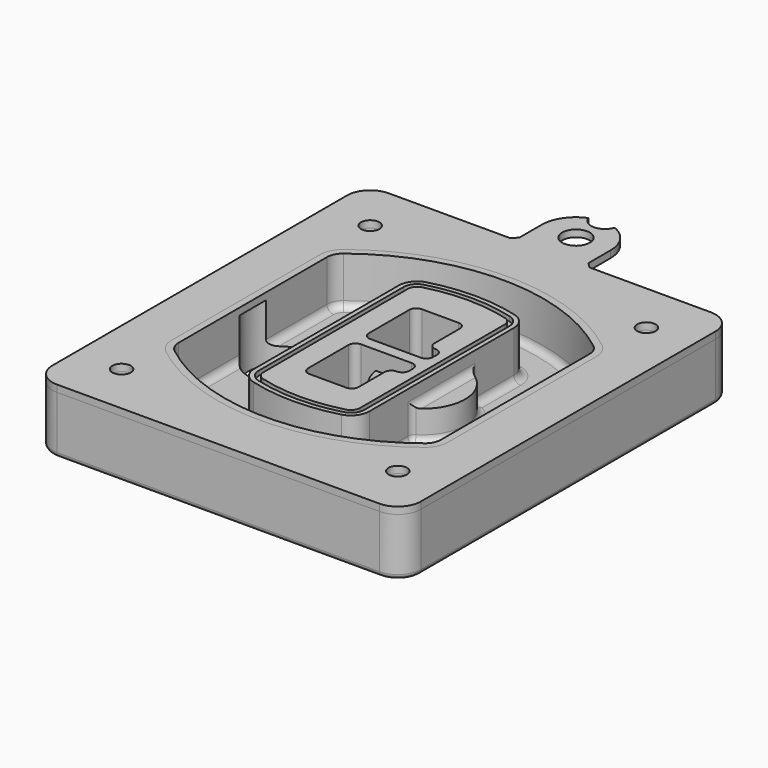
from build123d import *

# Parameters (mm, degrees)
F0_R      = 4
F1_DEPTH  = 25
F2_DEPTH  = 3
F3_DEPTH  = 18
F5_DEPTH  = 21
F6_DEPTH  = 2
F8_DEPTH  = 20
F9_DEPTH  = 16
F10_DEPTH = 25
F7_R      = 6
F7_R_2    = 4
F11_DEPTH = 6
F13_DEPTH = 9
F14_R     = 3
F15_R     = 2
F16_R     = 6
F16_R_2   = 4
F17_DEPTH = 3


with BuildPart() as f1:
    # F0 (on Top) → F1 (new body)
    with BuildSketch(Plane.XY):
        with BuildLine():
            ThreePointArc((-80, -80), (-77.0710678119, -87.0710678119), (-70, -90))
            Line((-70, -90), (70, -90))
            ThreePointArc((70, -90), (77.0710678119, -87.0710678119), (80, -80))
            Line((80, -80), (80, 80))
            ThreePointArc((80, 80), (77.0710678119, 87.0710678119), (70, 90))
            Line((70, 90), (-70, 90))
            ThreePointArc((-70, 90), (-77.0710678119, 87.0710678119), (-80, 80))
            Line((-80, 80), (-80, -80))
        make_face()
        with Locations((-60, -67.5)):
            Circle(F0_R, mode=Mode.SUBTRACT)
        with Locations((60, -67.5)):
            Circle(F0_R, mode=Mode.SUBTRACT)
        with Locations((-60, 67.5)):
            Circle(F0_R, mode=Mode.SUBTRACT)
        with BuildLine():
            ThreePointArc((-64, 40.2934422872), (-62.5820384798, 46.4328484224), (-58.6153846154, 51.3286200352))
            ThreePointArc((-58.6153846154, 51.3286200352), (0, 71.5), (58.6153846154, 51.3286200352))
            ThreePointArc((58.6153846154, 51.3286200352), (62.5820384798, 46.4328484224), (64, 40.2934422872))
            Line((64, 40.2934422872), (64, -40.2934422872))
            ThreePointArc((64, -40.2934422872), (62.5820384798, -46.4328484224), (58.6153846154, -51.3286200352))
            ThreePointArc((58.6153846154, -51.3286200352), (0, -71.5), (-58.6153846154, -51.3286200352))
            ThreePointArc((-58.6153846154, -51.3286200352), (-62.5820384798, -46.4328484224), (-64, -40.2934422872))
            Line((-64, -40.2934422872), (-64, 40.2934422872))
        make_face(mode=Mode.SUBTRACT)
        with Locations((60, 67.5)):
            Circle(F0_R, mode=Mode.SUBTRACT)
        with BuildLine():
            ThreePointArc((58.6153846154, 51.3286200352), (0, 71.5), (-58.6153846154, 51.3286200352))
            ThreePointArc((-58.6153846154, 51.3286200352), (-62.5820384798, 46.4328484224), (-64, 40.2934422872))
            Line((-64, 40.2934422872), (-64, -40.2934422872))
            ThreePointArc((-64, -40.2934422872), (-62.5820384798, -46.4328484224), (-58.6153846154, -51.3286200352))
            ThreePointArc((-58.6153846154, -51.3286200352), (0, -71.5), (58.6153846154, -51.3286200352))
            ThreePointArc((58.6153846154, -51.3286200352), (62.5820384798, -46.4328484224), (64, -40.2934422872))
            Line((64, -40.2934422872), (64, 40.2934422872))
            ThreePointArc((64, 40.2934422872), (62.5820384798, 46.4328484224), (58.6153846154, 51.3286200352))
        make_face()
        with BuildLine():
            Line((-60, -40.2934422872), (-60, 40.2934422872))
            ThreePointArc((-60, 40.2934422872), (-58.9871703427, 44.6787323838), (-56.1538461538, 48.1757121072))
            ThreePointArc((-56.1538461538, 48.1757121072), (0, 67.5), (56.1538461538, 48.1757121072))
            ThreePointArc((56.1538461538, 48.1757121072), (58.9871703427, 44.6787323838), (60, 40.2934422872))
            Line((60, 40.2934422872), (60, -40.2934422872))
            ThreePointArc((60, -40.2934422872), (58.9871703427, -44.6787323838), (56.1538461538, -48.1757121072))
            ThreePointArc((56.1538461538, -48.1757121072), (0, -67.5), (-56.1538461538, -48.1757121072))
            ThreePointArc((-56.1538461538, -48.1757121072), (-58.9871703427, -44.6787323838), (-60, -40.2934422872))
        make_face(mode=Mode.SUBTRACT)
        with BuildLine():
            ThreePointArc((-56.1538461538, 48.1757121072), (-58.9871703427, 44.6787323838), (-60, 40.2934422872))
            Line((-60, 40.2934422872), (-60, -40.2934422872))
            ThreePointArc((-60, -40.2934422872), (-58.9871703427, -44.6787323838), (-56.1538461538, -48.1757121072))
            ThreePointArc((-56.1538461538, -48.1757121072), (0, -67.5), (56.1538461538, -48.1757121072))
            ThreePointArc((56.1538461538, -48.1757121072), (58.9871703427, -44.6787323838), (60, -40.2934422872))
            Line((60, -40.2934422872), (60, 40.2934422872))
            ThreePointArc((60, 40.2934422872), (58.9871703427, 44.6787323838), (56.1538461538, 48.1757121072))
            ThreePointArc((56.1538461538, 48.1757121072), (0, 67.5), (-56.1538461538, 48.1757121072))
        make_face()
        with BuildLine():
            ThreePointArc((54.3076923077, 45.8110311612), (56.2910192399, 43.3631453548), (57, 40.2934422872))
            Line((57, 40.2934422872), (57, -40.2934422872))
            ThreePointArc((57, -40.2934422872), (56.2910192399, -43.3631453548), (54.3076923077, -45.8110311612))
            ThreePointArc((54.3076923077, -45.8110311612), (0, -64.5), (-54.3076923077, -45.8110311612))
            ThreePointArc((-54.3076923077, -45.8110311612), (-56.2910192399, -43.3631453548), (-57, -40.2934422872))
            Line((-57, -40.2934422872), (-57, 40.2934422872))
            ThreePointArc((-57, 40.2934422872), (-56.2910192399, 43.3631453548), (-54.3076923077, 45.8110311612))
            ThreePointArc((-54.3076923077, 45.8110311612), (0, 64.5), (54.3076923077, 45.8110311612))
        make_face(mode=Mode.SUBTRACT)
        with BuildLine():
            Line((57, -40.2934422872), (57, 40.2934422872))
            ThreePointArc((57, 40.2934422872), (56.2910192399, 43.3631453548), (54.3076923077, 45.8110311612))
            ThreePointArc((54.3076923077, 45.8110311612), (0, 64.5), (-54.3076923077, 45.8110311612))
            ThreePointArc((-54.3076923077, 45.8110311612), (-56.2910192399, 43.3631453548), (-57, 40.2934422872))
            Line((-57, 40.2934422872), (-57, -40.2934422872))
            ThreePointArc((-57, -40.2934422872), (-56.2910192399, -43.3631453548), (-54.3076923077, -45.8110311612))
            ThreePointArc((-54.3076923077, -45.8110311612), (0, -64.5), (54.3076923077, -45.8110311612))
            ThreePointArc((54.3076923077, -45.8110311612), (56.2910192399, -43.3631453548), (57, -40.2934422872))
        make_face()
    extrude(amount=-F1_DEPTH)

    # F0 (on Top) → F2 (join)
    with BuildSketch(Plane.XY):
        with BuildLine():
            ThreePointArc((-56.1538461538, 48.1757121072), (-58.9871703427, 44.6787323838), (-60, 40.2934422872))
            Line((-60, 40.2934422872), (-60, -40.2934422872))
            ThreePointArc((-60, -40.2934422872), (-58.9871703427, -44.6787323838), (-56.1538461538, -48.1757121072))
            ThreePointArc((-56.1538461538, -48.1757121072), (0, -67.5), (56.1538461538, -48.1757121072))
            ThreePointArc((56.1538461538, -48.1757121072), (58.9871703427, -44.6787323838), (60, -40.2934422872))
            Line((60, -40.2934422872), (60, 40.2934422872))
            ThreePointArc((60, 40.2934422872), (58.9871703427, 44.6787323838), (56.1538461538, 48.1757121072))
            ThreePointArc((56.1538461538, 48.1757121072), (0, 67.5), (-56.1538461538, 48.1757121072))
        make_face()
        with BuildLine():
            ThreePointArc((54.3076923077, 45.8110311612), (56.2910192399, 43.3631453548), (57, 40.2934422872))
            Line((57, 40.2934422872), (57, -40.2934422872))
            ThreePointArc((57, -40.2934422872), (56.2910192399, -43.3631453548), (54.3076923077, -45.8110311612))
            ThreePointArc((54.3076923077, -45.8110311612), (0, -64.5), (-54.3076923077, -45.8110311612))
            ThreePointArc((-54.3076923077, -45.8110311612), (-56.2910192399, -43.3631453548), (-57, -40.2934422872))
            Line((-57, -40.2934422872), (-57, 40.2934422872))
            ThreePointArc((-57, 40.2934422872), (-56.2910192399, 43.3631453548), (-54.3076923077, 45.8110311612))
            ThreePointArc((-54.3076923077, 45.8110311612), (0, 64.5), (54.3076923077, 45.8110311612))
        make_face(mode=Mode.SUBTRACT)
    extrude(amount=F2_DEPTH)

    # F0 (on Top) → F3 (cut)
    with BuildSketch(Plane.XY):
        with BuildLine():
            Line((57, -40.2934422872), (57, 40.2934422872))
            ThreePointArc((57, 40.2934422872), (56.2910192399, 43.3631453548), (54.3076923077, 45.8110311612))
            ThreePointArc((54.3076923077, 45.8110311612), (0, 64.5), (-54.3076923077, 45.8110311612))
            ThreePointArc((-54.3076923077, 45.8110311612), (-56.2910192399, 43.3631453548), (-57, 40.2934422872))
            Line((-57, 40.2934422872), (-57, -40.2934422872))
            ThreePointArc((-57, -40.2934422872), (-56.2910192399, -43.3631453548), (-54.3076923077, -45.8110311612))
            ThreePointArc((-54.3076923077, -45.8110311612), (0, -64.5), (54.3076923077, -45.8110311612))
            ThreePointArc((54.3076923077, -45.8110311612), (56.2910192399, -43.3631453548), (57, -40.2934422872))
        make_face()
    extrude(amount=-F3_DEPTH, mode=Mode.SUBTRACT)

    # F4 (on face) → F5 (join, through all)
    with BuildSketch(Plane.XY.offset(3)):
        with BuildLine():
            ThreePointArc((-25, -39.2465276821), (-23.3511545998, -44.1109737193), (-19.0842911877, -46.9702398883))
            ThreePointArc((-19.0842911877, -46.9702398883), (0, -49.5), (19.0842911877, -46.9702398883))
            ThreePointArc((19.0842911877, -46.9702398883), (23.3511545998, -44.1109737193), (25, -39.2465276821))
            Line((25, -39.2465276821), (25, 39.2465276821))
            ThreePointArc((25, 39.2465276821), (23.3511545998, 44.1109737193), (19.0842911877, 46.9702398883))
            ThreePointArc((19.0842911877, 46.9702398883), (0, 49.5), (-19.0842911877, 46.9702398883))
            ThreePointArc((-19.0842911877, 46.9702398883), (-23.3511545998, 44.1109737193), (-25, 39.2465276821))
            Line((-25, 39.2465276821), (-25, -39.2465276821))
        make_face()
        with BuildLine():
            ThreePointArc((18.5632183908, 45.0393118368), (21.7633659499, 42.89486221), (23, 39.2465276821))
            Line((23, 39.2465276821), (23, -39.2465276821))
            ThreePointArc((23, -39.2465276821), (21.7633659499, -42.89486221), (18.5632183908, -45.0393118368))
            ThreePointArc((18.5632183908, -45.0393118368), (0, -47.5), (-18.5632183908, -45.0393118368))
            ThreePointArc((-18.5632183908, -45.0393118368), (-21.7633659499, -42.89486221), (-23, -39.2465276821))
            Line((-23, -39.2465276821), (-23, 39.2465276821))
            ThreePointArc((-23, 39.2465276821), (-21.7633659499, 42.89486221), (-18.5632183908, 45.0393118368))
            ThreePointArc((-18.5632183908, 45.0393118368), (0, 47.5), (18.5632183908, 45.0393118368))
        make_face(mode=Mode.SUBTRACT)
        with BuildLine():
            Line((23, -39.2465276821), (23, 39.2465276821))
            ThreePointArc((23, 39.2465276821), (21.7633659499, 42.89486221), (18.5632183908, 45.0393118368))
            ThreePointArc((18.5632183908, 45.0393118368), (0, 47.5), (-18.5632183908, 45.0393118368))
            ThreePointArc((-18.5632183908, 45.0393118368), (-21.7633659499, 42.89486221), (-23, 39.2465276821))
            Line((-23, 39.2465276821), (-23, -39.2465276821))
            ThreePointArc((-23, -39.2465276821), (-21.7633659499, -42.89486221), (-18.5632183908, -45.0393118368))
            ThreePointArc((-18.5632183908, -45.0393118368), (0, -47.5), (18.5632183908, -45.0393118368))
            ThreePointArc((18.5632183908, -45.0393118368), (21.7633659499, -42.89486221), (23, -39.2465276821))
        make_face()
        with BuildLine():
            ThreePointArc((18.0421455939, 43.1083837852), (20.1755772999, 41.6787507007), (21, 39.2465276821))
            Line((21, 39.2465276821), (21, -39.2465276821))
            ThreePointArc((21, -39.2465276821), (20.1755772999, -41.6787507007), (18.0421455939, -43.1083837852))
            ThreePointArc((18.0421455939, -43.1083837852), (0, -45.5), (-18.0421455939, -43.1083837852))
            ThreePointArc((-18.0421455939, -43.1083837852), (-20.1755772999, -41.6787507007), (-21, -39.2465276821))
            Line((-21, -39.2465276821), (-21, 39.2465276821))
            ThreePointArc((-21, 39.2465276821), (-20.1755772999, 41.6787507007), (-18.0421455939, 43.1083837852))
            ThreePointArc((-18.0421455939, 43.1083837852), (0, 45.5), (18.0421455939, 43.1083837852))
        make_face(mode=Mode.SUBTRACT)
        with BuildLine():
            Line((21, -39.2465276821), (21, 39.2465276821))
            ThreePointArc((21, 39.2465276821), (20.1755772999, 41.6787507007), (18.0421455939, 43.1083837852))
            ThreePointArc((18.0421455939, 43.1083837852), (0, 45.5), (-18.0421455939, 43.1083837852))
            ThreePointArc((-18.0421455939, 43.1083837852), (-20.1755772999, 41.6787507007), (-21, 39.2465276821))
            Line((-21, 39.2465276821), (-21, -39.2465276821))
            ThreePointArc((-21, -39.2465276821), (-20.1755772999, -41.6787507007), (-18.0421455939, -43.1083837852))
            ThreePointArc((-18.0421455939, -43.1083837852), (0, -45.5), (18.0421455939, -43.1083837852))
            ThreePointArc((18.0421455939, -43.1083837852), (20.1755772999, -41.6787507007), (21, -39.2465276821))
        make_face()
        with BuildLine():
            Line((-8, -2.5), (14, -2.5))
            ThreePointArc((14, -2.5), (16.1213203436, -3.3786796564), (17, -5.5))
            Line((17, -5.5), (17, -7.5))
            ThreePointArc((17, -7.5), (16.1213203436, -9.6213203436), (14, -10.5))
            ThreePointArc((14, -10.5), (11.8786796564, -11.3786796564), (11, -13.5))
            Line((11, -13.5), (11, -27.5))
            ThreePointArc((11, -27.5), (10.1213203436, -29.6213203436), (8, -30.5))
            Line((8, -30.5), (-8, -30.5))
            ThreePointArc((-8, -30.5), (-10.1213203436, -29.6213203436), (-11, -27.5))
            Line((-11, -27.5), (-11, -5.5))
            ThreePointArc((-11, -5.5), (-10.1213203436, -3.3786796564), (-8, -2.5))
        make_face(mode=Mode.SUBTRACT)
        with BuildLine():
            ThreePointArc((-8, 2.5), (-10.1213203436, 3.3786796564), (-11, 5.5))
            Line((-11, 5.5), (-11, 27.5))
            ThreePointArc((-11, 27.5), (-10.1213203436, 29.6213203436), (-8, 30.5))
            Line((-8, 30.5), (8, 30.5))
            ThreePointArc((8, 30.5), (10.1213203436, 29.6213203436), (11, 27.5))
            Line((11, 27.5), (11, 13.5))
            ThreePointArc((11, 13.5), (11.8786796564, 11.3786796564), (14, 10.5))
            ThreePointArc((14, 10.5), (16.1213203436, 9.6213203436), (17, 7.5))
            Line((17, 7.5), (17, 5.5))
            ThreePointArc((17, 5.5), (16.1213203436, 3.3786796564), (14, 2.5))
            Line((14, 2.5), (-8, 2.5))
        make_face(mode=Mode.SUBTRACT)
    extrude(amount=-F5_DEPTH)

    # F4 (on face) → F6 (cut)
    with BuildSketch(Plane.XY.offset(3)):
        with BuildLine():
            Line((23, -39.2465276821), (23, 39.2465276821))
            ThreePointArc((23, 39.2465276821), (21.7633659499, 42.89486221), (18.5632183908, 45.0393118368))
            ThreePointArc((18.5632183908, 45.0393118368), (0, 47.5), (-18.5632183908, 45.0393118368))
            ThreePointArc((-18.5632183908, 45.0393118368), (-21.7633659499, 42.89486221), (-23, 39.2465276821))
            Line((-23, 39.2465276821), (-23, -39.2465276821))
            ThreePointArc((-23, -39.2465276821), (-21.7633659499, -42.89486221), (-18.5632183908, -45.0393118368))
            ThreePointArc((-18.5632183908, -45.0393118368), (0, -47.5), (18.5632183908, -45.0393118368))
            ThreePointArc((18.5632183908, -45.0393118368), (21.7633659499, -42.89486221), (23, -39.2465276821))
        make_face()
        with BuildLine():
            ThreePointArc((18.0421455939, 43.1083837852), (20.1755772999, 41.6787507007), (21, 39.2465276821))
            Line((21, 39.2465276821), (21, -39.2465276821))
            ThreePointArc((21, -39.2465276821), (20.1755772999, -41.6787507007), (18.0421455939, -43.1083837852))
            ThreePointArc((18.0421455939, -43.1083837852), (0, -45.5), (-18.0421455939, -43.1083837852))
            ThreePointArc((-18.0421455939, -43.1083837852), (-20.1755772999, -41.6787507007), (-21, -39.2465276821))
            Line((-21, -39.2465276821), (-21, 39.2465276821))
            ThreePointArc((-21, 39.2465276821), (-20.1755772999, 41.6787507007), (-18.0421455939, 43.1083837852))
            ThreePointArc((-18.0421455939, 43.1083837852), (0, 45.5), (18.0421455939, 43.1083837852))
        make_face(mode=Mode.SUBTRACT)
    extrude(amount=-F6_DEPTH, mode=Mode.SUBTRACT)

    # F7 (on face) → F8 (join)
    with BuildSketch(Plane(origin=(0, 0, -25), x_dir=(1, 0, 0), z_dir=(0, 0, -1))):
        with BuildLine():
            ThreePointArc((3.28842436, 0), (16.7567035675, 13.4682792075), (30.224982775, 0))
            Line((30.224982775, 0), (35.224982775, 0))
            ThreePointArc((35.224982775, 0), (16.7567035675, 18.4682792075), (-1.71157564, 0))
            Line((-1.71157564, 0), (3.28842436, 0))
        make_face()
        with BuildLine():
            Line((3.28842436, 0), (30.224982775, 0))
            ThreePointArc((30.224982775, 0), (16.7567035675, 13.4682792075), (3.28842436, 0))
        make_face()
        with BuildLine():
            ThreePointArc((3.28842436, 0), (16.7567035675, -13.4682792075), (30.224982775, 0))
            Line((30.224982775, 0), (3.28842436, 0))
        make_face()
        with BuildLine():
            Line((35.224982775, 0), (30.224982775, 0))
            ThreePointArc((30.224982775, 0), (16.7567035675, -13.4682792075), (3.28842436, 0))
            Line((3.28842436, 0), (-1.71157564, 0))
            ThreePointArc((-1.71157564, 0), (16.7567035675, -18.4682792075), (35.224982775, 0))
        make_face()
    extrude(amount=-F8_DEPTH)

    # F7 (on face) → F9 (cut)
    with BuildSketch(Plane(origin=(0, 0, -25), x_dir=(1, 0, 0), z_dir=(0, 0, -1))):
        with BuildLine():
            Line((3.28842436, 0), (30.224982775, 0))
            ThreePointArc((30.224982775, 0), (16.7567035675, 13.4682792075), (3.28842436, 0))
        make_face()
        with BuildLine():
            ThreePointArc((3.28842436, 0), (16.7567035675, -13.4682792075), (30.224982775, 0))
            Line((30.224982775, 0), (3.28842436, 0))
        make_face()
    extrude(amount=-F9_DEPTH, mode=Mode.SUBTRACT)

    # F7 (on face) → F10 (cut)
    with BuildSketch(Plane(origin=(0, 0, -25), x_dir=(1, 0, 0), z_dir=(0, 0, -1))):
        with BuildLine():
            Line((-59.0318229325, 0), (-32.0952645175, 0))
            ThreePointArc((-32.0952645175, 0), (-45.563543725, 13.4682792075), (-59.0318229325, 0))
        make_face()
        with BuildLine():
            ThreePointArc((-59.0318229325, 0), (-45.563543725, -13.4682792075), (-32.0952645175, 0))
            Line((-32.0952645175, 0), (-59.0318229325, 0))
        make_face()
    extrude(amount=-F10_DEPTH, mode=Mode.SUBTRACT)

    # F7 (on face) → F11 (cut)
    with BuildSketch(Plane(origin=(0, 0, -25), x_dir=(1, 0, 0), z_dir=(0, 0, -1))):
        with Locations((60, -67.5)):
            Circle(F7_R)
        with Locations((60, -67.5)):
            Circle(F7_R_2, mode=Mode.SUBTRACT)
        with Locations((-60, -67.5)):
            Circle(F7_R)
        with Locations((-60, -67.5)):
            Circle(F7_R_2, mode=Mode.SUBTRACT)
        with Locations((-60, 67.5)):
            Circle(F7_R)
        with Locations((-60, 67.5)):
            Circle(F7_R_2, mode=Mode.SUBTRACT)
        with Locations((60, 67.5)):
            Circle(F7_R)
        with Locations((60, 67.5)):
            Circle(F7_R_2, mode=Mode.SUBTRACT)
    extrude(amount=-F11_DEPTH, mode=Mode.SUBTRACT)

    # F12 (on face) → F13 (cut, through all)
    with BuildSketch(Plane(origin=(0, 0, -9), x_dir=(1, 0, 0), z_dir=(0, 0, -1))):
        with BuildLine():
            Line((11, 13.5), (11, 17.5481537753))
            ThreePointArc((11, 17.5481537753), (2.5696536419, 11.8239143813), (-1.5415842455, 2.5))
            Line((-1.5415842455, 2.5), (3.5224848595, 2.5))
            ThreePointArc((3.5224848595, 2.5), (6.1857188154, 8.3455872281), (11.2536447004, 12.2927168648))
            ThreePointArc((11.2536447004, 12.2927168648), (11.0640958889, 12.8831798879), (11, 13.5))
        make_face()
        with BuildLine():
            ThreePointArc((11.2536447004, -12.2927168648), (6.1857188154, -8.3455872281), (3.5224848595, -2.5))
            Line((3.5224848595, -2.5), (-1.5415842455, -2.5))
            ThreePointArc((-1.5415842455, -2.5), (2.5696536419, -11.8239143813), (11, -17.5481537753))
            Line((11, -17.5481537753), (11, -13.5))
            ThreePointArc((11, -13.5), (11.0640958889, -12.8831798879), (11.2536447004, -12.2927168648))
        make_face()
        with BuildLine():
            ThreePointArc((11.2536447004, 12.2927168648), (6.1857188154, 8.3455872281), (3.5224848595, 2.5))
            Line((3.5224848595, 2.5), (14, 2.5))
            ThreePointArc((14, 2.5), (16.1213203436, 3.3786796564), (17, 5.5))
            Line((17, 5.5), (17, 7.5))
            ThreePointArc((17, 7.5), (16.1213203436, 9.6213203436), (14, 10.5))
            ThreePointArc((14, 10.5), (12.3601599782, 10.9878446101), (11.2536447004, 12.2927168648))
        make_face()
        with BuildLine():
            Line((14, -2.5), (3.5224848595, -2.5))
            ThreePointArc((3.5224848595, -2.5), (6.1857188154, -8.3455872281), (11.2536447004, -12.2927168648))
            ThreePointArc((11.2536447004, -12.2927168648), (12.3601599782, -10.9878446101), (14, -10.5))
            ThreePointArc((14, -10.5), (16.1213203436, -9.6213203436), (17, -7.5))
            Line((17, -7.5), (17, -5.5))
            ThreePointArc((17, -5.5), (16.1213203436, -3.3786796564), (14, -2.5))
        make_face()
    extrude(amount=F13_DEPTH, mode=Mode.SUBTRACT)

    # F14
    f14_edges = [f1.edges().sort_by_distance(p)[0] for p in [
        (-57, -23.703476, -18),
        (-57, 23.703476, -18),
        (25, 0, -5),
        (25, 16.526506, -11.5),
        (25, -16.526506, -11.5),
        (25, -27.886517, -18),
        (35.224983, 0, -18),
        (23.351155, -44.110974, -18),
        (0, -64.5, -18),
        (-56.291019, -43.363145, -18),
        (-56.291019, 43.363145, -18),
        (0, 64.5, -18),
        (56.291019, 43.363145, -18),
        (57, 0, -18),
        (56.291019, -43.363145, -18),
        (-23.351155, 44.110974, -18),
        (0, 49.5, -18),
        (-25, 0, -18),
        (23.351155, 44.110974, -18),
        (-23.351155, -44.110974, -18),
        (25, 27.886517, -18),
        (0, -49.5, -18),
    ]]
    fillet(f14_edges, radius=F14_R)

    # F15
    f15_edges = [f1.edges().sort_by_distance(p)[0] for p in [
        (0, -90, -25),
        (-77.071068, -87.071068, -25),
        (-80, 0, -25),
        (-77.071068, 87.071068, -25),
        (77.071068, -87.071068, -25),
        (0, 90, -25),
        (80, 0, -25),
        (77.071068, 87.071068, -25),
    ]]
    fillet(f15_edges, radius=F15_R)


with BuildPart() as f17:
    # F16 (on face) → F17 (new body, through all)
    with BuildSketch(Plane.XY):
        with BuildLine():
            ThreePointArc((5.6995065576, 118.125), (0, 114), (-5.6995065576, 118.125))
            ThreePointArc((-5.6995065576, 118.125), (-12.4597872848, 112.6018681035), (-15, 104.25))
            Line((-15, 104.25), (-15, 92.25))
            Line((-15, 92.25), (-17.25, 90))
            Line((-17.25, 90), (17.25, 90))
            Line((17.25, 90), (15, 92.25))
            Line((15, 92.25), (15, 104.25))
            ThreePointArc((15, 104.25), (12.4597872848, 112.6018681035), (5.6995065576, 118.125))
        make_face()
        with Locations((0, 104.25)):
            Circle(F16_R, mode=Mode.SUBTRACT)
        with BuildLine():
            Line((17.25, 90), (-17.25, 90))
            Line((-17.25, 90), (-70, 90))
            ThreePointArc((-70, 90), (-77.0710678119, 87.0710678119), (-80, 80))
            Line((-80, 80), (-80, -80))
            ThreePointArc((-80, -80), (-77.0710678119, -87.0710678119), (-70, -90))
            Line((-70, -90), (-17.25, -90))
            Line((-17.25, -90), (33, -90))
            Line((33, -90), (70, -90))
            ThreePointArc((70, -90), (77.0710678119, -87.0710678119), (80, -80))
            Line((80, -80), (80, 80))
            ThreePointArc((80, 80), (77.0710678119, 87.0710678119), (70, 90))
            Line((70, 90), (33, 90))
            Line((33, 90), (17.25, 90))
        make_face()
        with Locations((-60, -67.5)):
            Circle(F16_R_2, mode=Mode.SUBTRACT)
        with Locations((60, -67.5)):
            Circle(F16_R_2, mode=Mode.SUBTRACT)
        with Locations((-60, 67.5)):
            Circle(F16_R_2, mode=Mode.SUBTRACT)
        with BuildLine():
            ThreePointArc((-60, 40.2934422872), (-58.9871703427, 44.6787323838), (-56.1538461538, 48.1757121072))
            ThreePointArc((-56.1538461538, 48.1757121072), (0, 67.5), (56.1538461538, 48.1757121072))
            ThreePointArc((56.1538461538, 48.1757121072), (58.9871703427, 44.6787323838), (60, 40.2934422872))
            Line((60, 40.2934422872), (60, -40.2934422872))
            ThreePointArc((60, -40.2934422872), (58.9871703427, -44.6787323838), (56.1538461538, -48.1757121072))
            ThreePointArc((56.1538461538, -48.1757121072), (0, -67.5), (-56.1538461538, -48.1757121072))
            ThreePointArc((-56.1538461538, -48.1757121072), (-58.9871703427, -44.6787323838), (-60, -40.2934422872))
            Line((-60, -40.2934422872), (-60, 40.2934422872))
        make_face(mode=Mode.SUBTRACT)
        with Locations((60, 67.5)):
            Circle(F16_R_2, mode=Mode.SUBTRACT)
    extrude(amount=F17_DEPTH)


solid = Compound([f1.part, f17.part])
